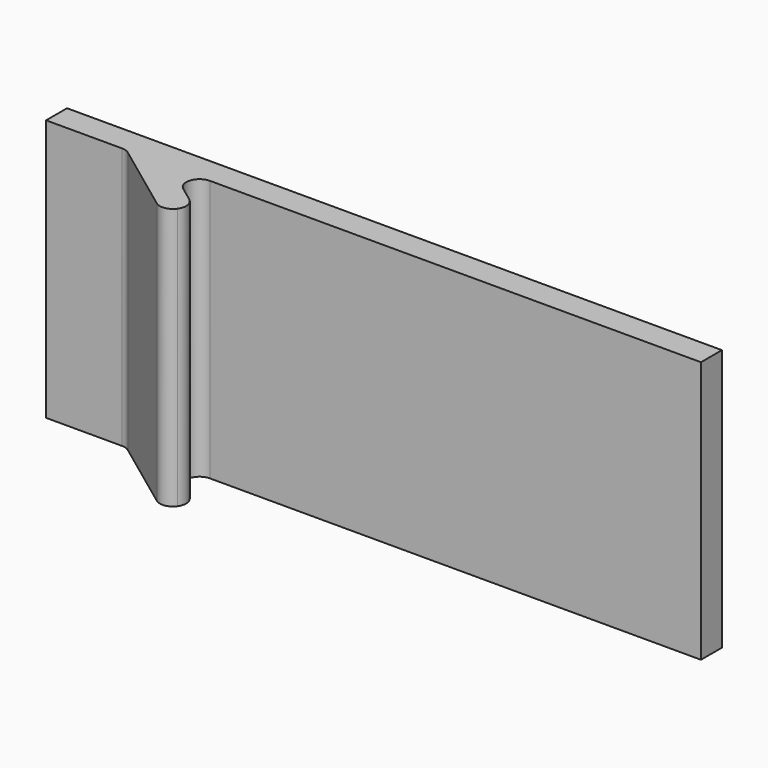
from build123d import *

# Parameters (mm, degrees)
F0_W     = 250
F0_H     = 100
F1_DEPTH = 5
F4_DEPTH = 50
F5_R     = 5
F6_R     = 4.99999


# Not quite as in the source:
# - two fillets or chamfers of one size are made in one step
# - a fillet or chamfer is up to 0.001 mm smaller than in the source, because OpenCascade refuses the exact size


with BuildPart() as f1:
    # F0 (on Front) → F1 (new body, symmetric)
    with BuildSketch(Plane.XZ):
        Rectangle(F0_W, F0_H)
    extrude(amount=F1_DEPTH, both=True)

    # F3 (on Top) → F4 (join, symmetric)
    with BuildSketch(Plane.XY):
        Polygon((-55.8243768029, -21.1299679096), (-77.5685643683, -5), (-94.3532884121, -5), (-61.7821750806, -29.1614459605), align=None)
    extrude(amount=F4_DEPTH, both=True)

    # F5
    f5_edges = [f1.edges().sort_by_distance(p)[0] for p in [
        (-94.353288, -5, 0),
        (-77.568564, -5, 0),
    ]]
    fillet(f5_edges, radius=F5_R)

    # F6 (radius 5 in the source; OpenCascade refuses exactly that, so slightly less here)
    f6_edges = [f1.edges().sort_by_distance(p)[0] for p in [
        (-61.782175, -29.161446, 0),
        (-55.824377, -21.129968, 0),
    ]]
    fillet(f6_edges, radius=F6_R)


solid = f1.part
